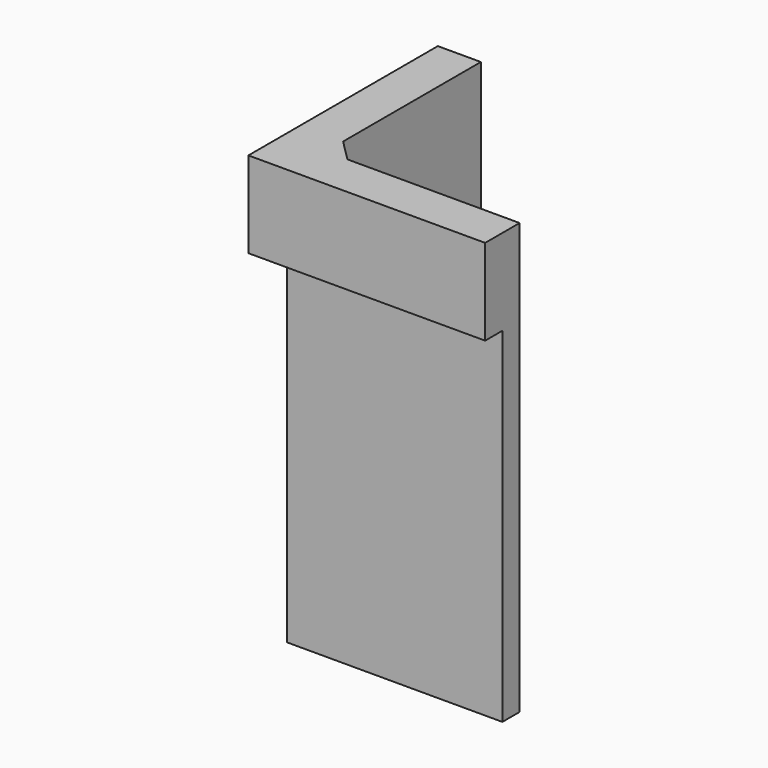
from build123d import *

# Parameters (mm, degrees)
F1_DEPTH = 63.5
F3_DEPTH = 12.7
F5_DEPTH = 31.75


# Not quite as in the source:
# - a pattern or mirror of a feature is missing from the dataset's text; its kind, count and spacing are read off the source's solid


with BuildPart() as f1:
    # F0 (on Top) → F1 (new body)
    with BuildSketch(Plane.XY):
        Polygon((0, 9.525), (0, 0), (9.525, 0), align=None)
    extrude(amount=F1_DEPTH)

    # F2 (on face) → F3 (join)
    with BuildSketch(Plane.XY.offset(63.5)):
        Polygon((12.7, -3.175), (4.7625, 4.7625), (-3.175, 12.7), (-3.175, -3.175), align=None)
    extrude(amount=-F3_DEPTH)

    # F4 (on face) → F5 (join)
    with BuildSketch(Plane.XZ):
        Polygon((0, 50.8), (0, 0), (3.175, 0), (3.175, 63.5), (-3.175, 63.5), (-3.175, 50.8), align=None)
    f5 = extrude(amount=-F5_DEPTH)

    # F5_copies: F5 across plane
    add(f5.mirror(Plane(origin=(0, 0, 0), x_dir=(-0.7071067812, -0.7071067812, 0), z_dir=(0.7071067812, -0.7071067812, 0))))


solid = f1.part
